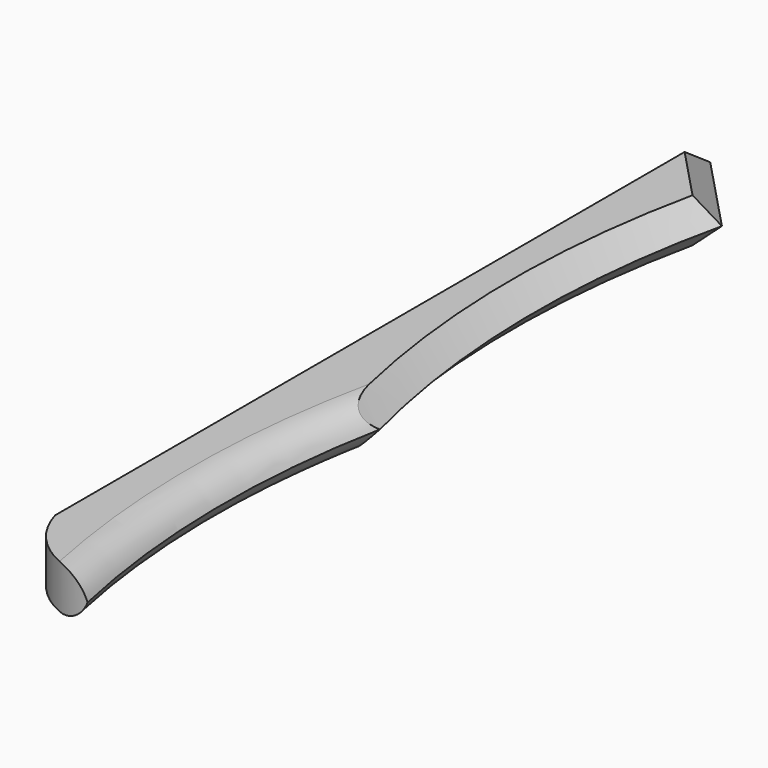
from build123d import *

# Parameters (mm, degrees)
F1_DEPTH    = 6.604
F2_T2_ANGLE = 37.6266885083
F2_T4_ANGLE = 37.6266885083
F3_T1_DEPTH = 39.1771149622
F4_T2_ANGLE = 30.7081908039
F4_T4_ANGLE = 30.7081908039


# Not quite as in the source:
# - a fillet or chamfer that OpenCascade refuses, or shapes differently, is made with other operations: its cross-section is extruded or revolved along the edge and cut away or added
# - ends of sketch curves that miss each other by under 0.0002 mm in the source are joined


with BuildPart() as f1:
    # F0 (on Top) → F1 (new body)
    with BuildSketch(Plane.XY):
        with BuildLine():
            Line((0, 76.2824639678), (0, 0))
            Line((0, 0), (13.1280263886, 0))
            ThreePointArc((13.1280263886, 0), (9.4882529844, 31.2224067748), (13.1280263886, 62.4448174897))
            Line((13.1280263886, 62.4448174897), (0, 76.2824639678))
        make_face()
        with BuildLine():
            Line((13.1280263886, 0), (0, 0))
            Line((0, 0), (0, -48.9660091698))
            ThreePointArc((0, -48.9660091698), (4.8963223511, -56.1371050306), (13.1280263886, -58.900732547))
            ThreePointArc((13.1280263886, -58.900732547), (9.9051564545, -29.4503682436), (13.1280263886, 0))
        make_face()
    extrude(amount=F1_DEPTH)

    # F2: chamfer of 5.08 on 2 edges, made by hand

    # F2_s1 → F2_t2 (revolve, cut)
    with BuildSketch(Plane(origin=(5.5719325615, -16.3549575283, 0), x_dir=(0, 0, 1), z_dir=(0.3224861622, -0.9465741784, 0))):
        Polygon((1.524, -11.7983946988), (6.604, -6.7183946988), (6.604, -11.7983946988), align=None)
    revolve(axis=Axis((145.2229057415, 31.2224087449, 6.604), (0, 0, -1)), revolution_arc=F2_T2_ANGLE, mode=Mode.SUBTRACT)

    # F2_s3 → F2_t4 (revolve, cut)
    with BuildSketch(Plane(origin=(5.5719325615, -16.3549575283, 0), x_dir=(0, 0, 1), z_dir=(0.3224861622, -0.9465741784, 0))):
        Polygon((5.08, -11.7983946988), (0, -6.7183946988), (0, -11.7983946988), align=None)
    revolve(axis=Axis((145.2229057415, 31.2224087449, 0), (0, 0, -1)), revolution_arc=F2_T4_ANGLE, mode=Mode.SUBTRACT)

    # F3: chamfer of 5.08 on 2 edges, made by hand

    # F3_s2 → F3_t1 (cut)
    with BuildSketch(Plane(origin=(-20.115918924, 21.2032613595, 0), x_dir=(0, 0, 1), z_dir=(-0.6882605094, 0.725463625, 0))):
        Polygon((5.08, 52.5022075061), (0, 47.4222075061), (0, 52.5022075061), align=None)
        Polygon((1.524, 52.5022075061), (6.604, 47.4222075061), (6.604, 52.5022075061), align=None)
    extrude(amount=F3_T1_DEPTH, mode=Mode.SUBTRACT)

    # F4: fillet of radius 5.08 on 2 edges, made by hand

    # F4_s1 → F4_t2 (revolve, cut)
    with BuildSketch(Plane(origin=(22.2878822439, -69.2757873609, 0), x_dir=(0, 0, 1), z_dir=(0.3062665426, -0.9519457994, 0))):
        with BuildLine():
            ThreePointArc((6.604, 11.2139897709), (5.1161024484, 7.6218873224), (1.524, 6.1339897709))
            Line((1.524, 6.1339897709), (6.604, 6.1339897709))
            Line((6.604, 6.1339897709), (6.604, 11.2139897709))
        make_face()
    revolve(axis=Axis((146.0743134808, -29.4503662735, 6.604), (0, 0, -1)), revolution_arc=F4_T2_ANGLE, mode=Mode.SUBTRACT)

    # F4_s3 → F4_t4 (revolve, cut)
    with BuildSketch(Plane(origin=(22.2878822439, -69.2757873609, 0), x_dir=(0, 0, 1), z_dir=(0.3062665426, -0.9519457994, 0))):
        with BuildLine():
            ThreePointArc((0, 11.2139897709), (1.4878975516, 7.6218873224), (5.08, 6.1339897709))
            Line((5.08, 6.1339897709), (0, 6.1339897709))
            Line((0, 6.1339897709), (0, 11.2139897709))
        make_face()
    revolve(axis=Axis((146.0743134808, -29.4503662735, 0), (0, 0, -1)), revolution_arc=F4_T4_ANGLE, mode=Mode.SUBTRACT)


solid = f1.part
